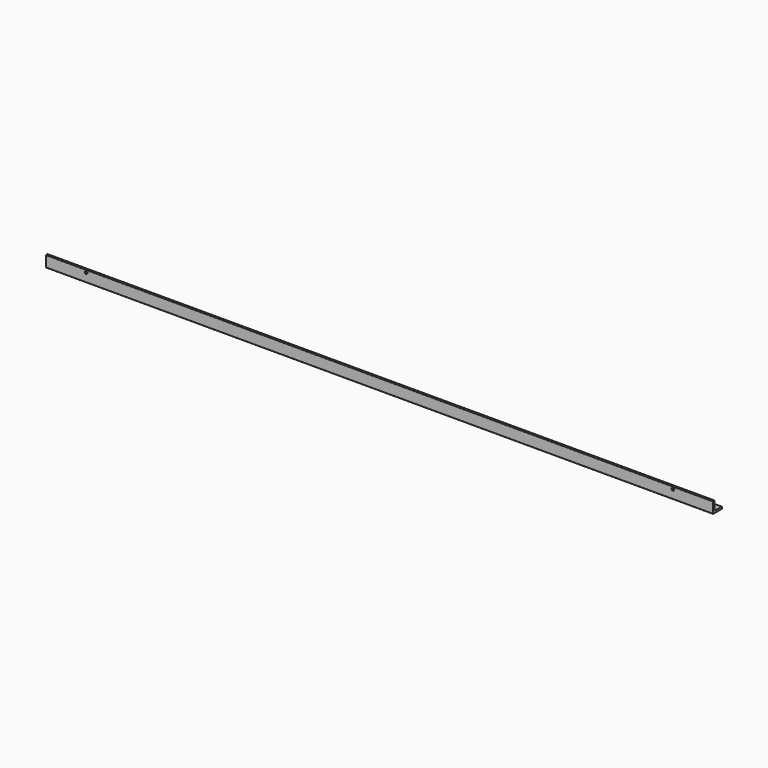
from build123d import *

# Parameters (mm, degrees)
F1_DEPTH = 750
F2_R     = 1
F3_R     = 2.38125
F4_R     = 2.5
F5_DEPTH = 25
F6_SIZE  = 0.5
F7_R     = 2.5
F8_DEPTH = 25
F9_SIZE  = 0.5


with BuildPart() as f1:
    # F0 (on Right) → F1 (new body, symmetric)
    with BuildSketch(Plane.YZ):
        Polygon((0, 25.4), (0, 0), (25.4, 0), (25.4, 4.7625), (4.7625, 4.7625), (4.7625, 25.4), align=None)
    extrude(amount=F1_DEPTH, both=True)

    # F2
    f2_edges = [f1.edges().sort_by_distance(p)[0] for p in [
        (0, 0, 25.4),
        (0, 4.7625, 25.4),
        (0, 0, 0),
        (0, 25.4, 4.7625),
        (0, 25.4, 0),
    ]]
    fillet(f2_edges, radius=F2_R)

    # F3
    f3_edges = [f1.edges().sort_by_distance(p)[0] for p in [
        (0, 4.7625, 4.7625),
    ]]
    fillet(f3_edges, radius=F3_R)

    # F4 (on face) → F5 (cut)
    with BuildSketch(Plane.XY.offset(4.7625)):
        with Locations((-730, 20)):
            Circle(F4_R)
        with Locations((0, 20)):
            Circle(F4_R)
        with Locations((730, 20)):
            Circle(F4_R)
    extrude(amount=-F5_DEPTH, mode=Mode.SUBTRACT)

    # F6
    f6_edges = [f1.edges().sort_by_distance(p)[0] for p in [
        (-732.5, 20, 4.7625),
        (-727.5, 20, 2.38125),
        (-732.5, 20, 0),
        (-2.5, 20, 4.7625),
        (2.5, 20, 2.38125),
        (-2.5, 20, 0),
        (727.5, 20, 4.7625),
        (732.5, 20, 2.38125),
        (727.5, 20, 0),
    ]]
    chamfer(f6_edges, length=F6_SIZE)

    # F7 (on face) → F8 (cut)
    with BuildSketch(Plane.XZ):
        with Locations((-660, 20)):
            Circle(F7_R)
        with Locations((660, 20)):
            Circle(F7_R)
    extrude(amount=-F8_DEPTH, mode=Mode.SUBTRACT)

    # F9
    f9_edges = [f1.edges().sort_by_distance(p)[0] for p in [
        (-662.5, 0, 20),
        (-657.5, 2.38125, 20),
        (-662.5, 4.7625, 20),
        (657.5, 0, 20),
        (662.5, 2.38125, 20),
        (657.5, 4.7625, 20),
    ]]
    chamfer(f9_edges, length=F9_SIZE)


solid = f1.part
